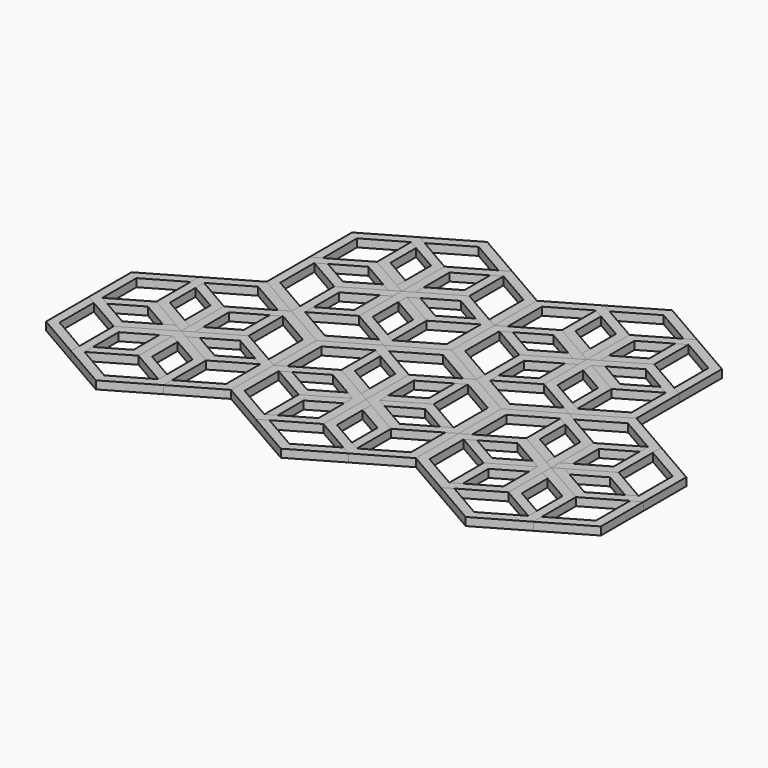
from build123d import *

# Parameters (mm, degrees)
F1_DEPTH = 1.5
F2_COUNT = 6
F3_COUNT = 3
F4_COUNT = 2
F4_ANGLE = 120


with BuildPart() as f1:
    # F0 (on Top) → F1 (new body)
    with BuildSketch(Plane.XY):
        Polygon((-8.6602540378, -5), (0, -10), (8.6602540378, -5), (8.6602540378, 5), (0, 10), (-8.6602540378, 5), align=None)
        Polygon((-6.9282032303, 4), (0, 8), (6.9282032303, 4), (6.9282032303, -4), (0, -8), (-6.9282032303, -4), align=None, mode=Mode.SUBTRACT)
    extrude(amount=F1_DEPTH)


with BuildPart() as f2_1:
    # F2: instance of F1
    add(f1.part.rotate(Axis((8.6602540378, 5, 0.75), (0, 0, -1)), 1 * 360 / F2_COUNT))


with BuildPart() as f2_2:
    # F2: instance of F1
    add(f1.part.rotate(Axis((8.6602540378, 5, 0.75), (0, 0, -1)), 2 * 360 / F2_COUNT))


with BuildPart() as f2_3:
    # F2: instance of F1
    add(f1.part.rotate(Axis((8.6602540378, 5, 0.75), (0, 0, -1)), 3 * 360 / F2_COUNT))


with BuildPart() as f2_4:
    # F2: instance of F1
    add(f1.part.rotate(Axis((8.6602540378, 5, 0.75), (0, 0, -1)), 4 * 360 / F2_COUNT))


with BuildPart() as f2_5:
    # F2: instance of F1
    add(f1.part.rotate(Axis((8.6602540378, 5, 0.75), (0, 0, -1)), 5 * 360 / F2_COUNT))


with BuildPart() as f3_1:
    # F3: instance of F1
    add(f1.part.rotate(Axis((25.9807621135, 15, 0.75), (0, 0, -1)), 1 * 360 / F3_COUNT))


with BuildPart() as f3_2:
    # F3: instance of F1
    add(f1.part.rotate(Axis((25.9807621135, 15, 0.75), (0, 0, -1)), 2 * 360 / F3_COUNT))


with BuildPart() as f3_3:
    # F3: instance of F2_1
    add(f2_1.part.rotate(Axis((25.9807621135, 15, 0.75), (0, 0, -1)), 1 * 360 / F3_COUNT))


with BuildPart() as f3_4:
    # F3: instance of F2_1
    add(f2_1.part.rotate(Axis((25.9807621135, 15, 0.75), (0, 0, -1)), 2 * 360 / F3_COUNT))


with BuildPart() as f3_5:
    # F3: instance of F2_5
    add(f2_5.part.rotate(Axis((25.9807621135, 15, 0.75), (0, 0, -1)), 1 * 360 / F3_COUNT))


with BuildPart() as f3_6:
    # F3: instance of F2_5
    add(f2_5.part.rotate(Axis((25.9807621135, 15, 0.75), (0, 0, -1)), 2 * 360 / F3_COUNT))


with BuildPart() as f3_7:
    # F3: instance of F2_4
    add(f2_4.part.rotate(Axis((25.9807621135, 15, 0.75), (0, 0, -1)), 1 * 360 / F3_COUNT))


with BuildPart() as f3_8:
    # F3: instance of F2_4
    add(f2_4.part.rotate(Axis((25.9807621135, 15, 0.75), (0, 0, -1)), 2 * 360 / F3_COUNT))


with BuildPart() as f3_9:
    # F3: instance of F2_3
    add(f2_3.part.rotate(Axis((25.9807621135, 15, 0.75), (0, 0, -1)), 1 * 360 / F3_COUNT))


with BuildPart() as f3_10:
    # F3: instance of F2_3
    add(f2_3.part.rotate(Axis((25.9807621135, 15, 0.75), (0, 0, -1)), 2 * 360 / F3_COUNT))


with BuildPart() as f3_11:
    # F3: instance of F2_2
    add(f2_2.part.rotate(Axis((25.9807621135, 15, 0.75), (0, 0, -1)), 1 * 360 / F3_COUNT))


with BuildPart() as f3_12:
    # F3: instance of F2_2
    add(f2_2.part.rotate(Axis((25.9807621135, 15, 0.75), (0, 0, -1)), 2 * 360 / F3_COUNT))


with BuildPart() as f4_1:
    # F4: instance of F1
    add(f1.part.rotate(Axis((8.6602540378, 25, 0.75), (0, 0, -1)), 1 * F4_ANGLE / (F4_COUNT - 1)))


with BuildPart() as f4_2:
    # F4: instance of F3_3
    add(f3_3.part.rotate(Axis((8.6602540378, 25, 0.75), (0, 0, -1)), 1 * F4_ANGLE / (F4_COUNT - 1)))


with BuildPart() as f4_3:
    # F4: instance of F2_1
    add(f2_1.part.rotate(Axis((8.6602540378, 25, 0.75), (0, 0, -1)), 1 * F4_ANGLE / (F4_COUNT - 1)))


with BuildPart() as f4_4:
    # F4: instance of F3_1
    add(f3_1.part.rotate(Axis((8.6602540378, 25, 0.75), (0, 0, -1)), 1 * F4_ANGLE / (F4_COUNT - 1)))


with BuildPart() as f4_5:
    # F4: instance of F2_5
    add(f2_5.part.rotate(Axis((8.6602540378, 25, 0.75), (0, 0, -1)), 1 * F4_ANGLE / (F4_COUNT - 1)))


with BuildPart() as f4_6:
    # F4: instance of F2_4
    add(f2_4.part.rotate(Axis((8.6602540378, 25, 0.75), (0, 0, -1)), 1 * F4_ANGLE / (F4_COUNT - 1)))


with BuildPart() as f4_7:
    # F4: instance of F2_3
    add(f2_3.part.rotate(Axis((8.6602540378, 25, 0.75), (0, 0, -1)), 1 * F4_ANGLE / (F4_COUNT - 1)))


with BuildPart() as f4_8:
    # F4: instance of F3_7
    add(f3_7.part.rotate(Axis((8.6602540378, 25, 0.75), (0, 0, -1)), 1 * F4_ANGLE / (F4_COUNT - 1)))


with BuildPart() as f4_9:
    # F4: instance of F3_9
    add(f3_9.part.rotate(Axis((8.6602540378, 25, 0.75), (0, 0, -1)), 1 * F4_ANGLE / (F4_COUNT - 1)))


with BuildPart() as f4_10:
    # F4: instance of F3_11
    add(f3_11.part.rotate(Axis((8.6602540378, 25, 0.75), (0, 0, -1)), 1 * F4_ANGLE / (F4_COUNT - 1)))


with BuildPart() as f4_11:
    # F4: instance of F2_2
    add(f2_2.part.rotate(Axis((8.6602540378, 25, 0.75), (0, 0, -1)), 1 * F4_ANGLE / (F4_COUNT - 1)))


with BuildPart() as f4_12:
    # F4: instance of F3_5
    add(f3_5.part.rotate(Axis((8.6602540378, 25, 0.75), (0, 0, -1)), 1 * F4_ANGLE / (F4_COUNT - 1)))


with BuildPart() as f4_13:
    # F4: instance of F3_2
    add(f3_2.part.rotate(Axis((8.6602540378, 25, 0.75), (0, 0, -1)), 1 * F4_ANGLE / (F4_COUNT - 1)))


with BuildPart() as f4_14:
    # F4: instance of F3_4
    add(f3_4.part.rotate(Axis((8.6602540378, 25, 0.75), (0, 0, -1)), 1 * F4_ANGLE / (F4_COUNT - 1)))


with BuildPart() as f4_15:
    # F4: instance of F3_12
    add(f3_12.part.rotate(Axis((8.6602540378, 25, 0.75), (0, 0, -1)), 1 * F4_ANGLE / (F4_COUNT - 1)))


with BuildPart() as f4_16:
    # F4: instance of F3_10
    add(f3_10.part.rotate(Axis((8.6602540378, 25, 0.75), (0, 0, -1)), 1 * F4_ANGLE / (F4_COUNT - 1)))


with BuildPart() as f4_17:
    # F4: instance of F3_8
    add(f3_8.part.rotate(Axis((8.6602540378, 25, 0.75), (0, 0, -1)), 1 * F4_ANGLE / (F4_COUNT - 1)))


with BuildPart() as f4_18:
    # F4: instance of F3_6
    add(f3_6.part.rotate(Axis((8.6602540378, 25, 0.75), (0, 0, -1)), 1 * F4_ANGLE / (F4_COUNT - 1)))


solid = Compound([f1.part, f2_1.part, f2_2.part, f2_3.part, f2_4.part, f2_5.part, f3_1.part, f3_2.part, f3_3.part, f3_4.part, f3_5.part, f3_6.part, f3_7.part, f3_8.part, f3_9.part, f3_10.part, f3_11.part, f3_12.part, f4_1.part, f4_2.part, f4_3.part, f4_4.part, f4_5.part, f4_6.part, f4_7.part, f4_8.part, f4_9.part, f4_10.part, f4_11.part, f4_12.part, f4_13.part, f4_14.part, f4_15.part, f4_16.part, f4_17.part, f4_18.part])
